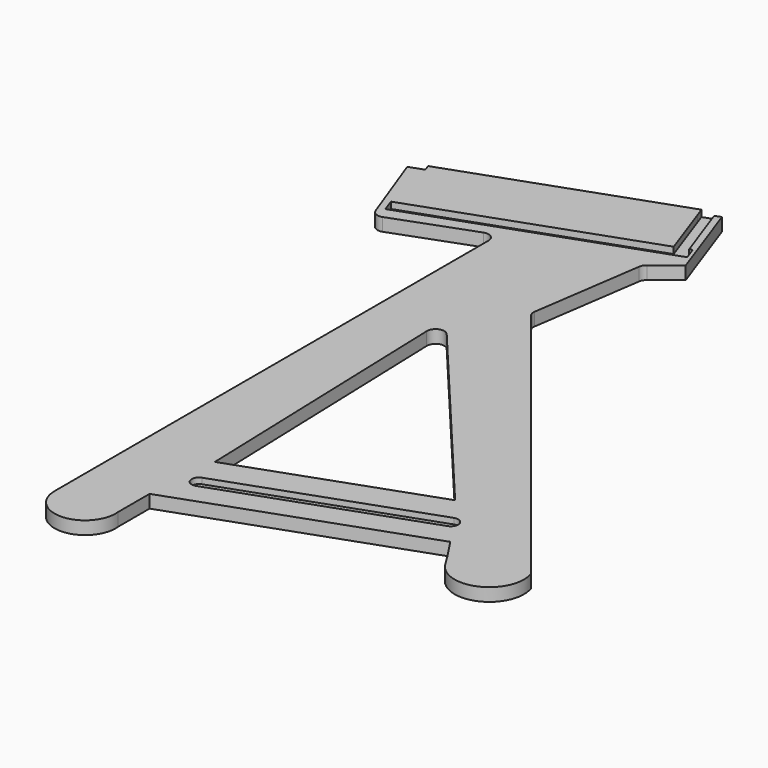
from build123d import *

# Parameters (mm, degrees)
F1_DEPTH = 19.05
F3_DEPTH = 8.4666582
F5_DEPTH = 9.525


# Not quite as in the source:
# - a feature names something its author has since deleted; it is built from what else it names


with BuildPart() as f1:
    # F0 (on Top) → F1 (new body)
    with BuildSketch(Plane.XY):
        with BuildLine():
            Line((727.2677384075, 427.9083177516), (727.2677384075, -283.5772421425))
            ThreePointArc((727.2677384075, -283.5772421425), (774.4074471785, -328.2362889839), (816.4554812019, -278.7535097314))
            Line((816.4554812019, -278.7535097314), (816.4554812019, -221.0955097314))
            Line((816.4554812019, -221.0955097314), (1159.4623036636, -98.9686407408))
            Line((1159.4623036636, -98.9686407408), (1178.6487772739, -128.0367093729))
            Line((1178.6487772739, -128.0367093729), (1189.3036458742, -145.3996676047))
            ThreePointArc((1189.3036458742, -145.3996676047), (1254.3589120262, -165.180351508), (1280.8355912672, -102.5508970465))
            Line((1280.8355912672, -102.5508970465), (881.2480453078, 396.8848219998))
            ThreePointArc((881.2480453078, 396.8848219998), (878.9075846932, 401.4943033077), (878.5980767553, 406.6546597539))
            Line((878.5980767553, 406.6546597539), (902.2401524871, 568.497452094))
            ThreePointArc((902.2401524871, 568.497452094), (903.8120375637, 573.0182606597), (906.9455405898, 576.6362285378))
            Line((906.9455405898, 576.6362285378), (941.9003890149, 604.1852707886))
            Line((941.9003890149, 604.1852707886), (899.3018677789, 723.8279303566))
            Line((899.3018677789, 723.8279303566), (891.7270738587, 721.1309406639))
            Line((891.7270738587, 721.1309406639), (888.532184766, 730.1041401315))
            Line((888.532184766, 730.1041401315), (557.8398737201, 612.361827435))
            Line((557.8398737201, 612.361827435), (561.0347628128, 603.3886279674))
            Line((561.0347628128, 603.3886279674), (540.3738890749, 596.0323666485))
            Line((540.3738890749, 596.0323666485), (579.8650741531, 488.7713005475))
            ThreePointArc((579.8650741531, 488.7713005475), (586.4584656719, 481.6292642269), (596.1708798397, 481.2413137672))
            Line((596.1708798397, 481.2413137672), (710.1798289544, 523.2169221936))
            ThreePointArc((710.1798289544, 523.2169221936), (721.8328450807, 521.7157540947), (727.2677384075, 511.2990259602))
            Line((727.2677384075, 511.2990259602), (727.2677384075, 427.9083177516))
        make_face()
        with BuildLine():
            Line((1099.3852571882, -15.0422832395), (825.3589785984, -112.6087723988))
            Line((825.3589785984, -112.6087723988), (812.2279623998, 291.9047427935))
            ThreePointArc((812.2279623998, 291.9047427935), (820.3847868922, 304.1789193457), (834.6503380579, 300.4798321914))
            Line((834.6503380579, 300.4798321914), (1099.3852571882, -15.0422832395))
        make_face(mode=Mode.SUBTRACT)
    extrude(amount=F1_DEPTH)

    # F2 (on face) → F3 (cut)
    with BuildSketch(Plane.XY.offset(19.05)):
        with BuildLine():
            ThreePointArc((838.451528287, -152.2525984903), (831.9027765287, -166.0430988586), (845.6932768971, -172.5918506169))
            Line((845.6932768971, -172.5918506169), (1132.8356598603, -70.3553996504))
            ThreePointArc((1132.8356598603, -70.3553996504), (1139.3844116185, -56.564899282), (1125.5939112501, -50.0161475238))
            Line((1125.5939112501, -50.0161475238), (838.451528287, -152.2525984903))
        make_face()
    extrude(amount=-F3_DEPTH, mode=Mode.SUBTRACT)

    # F4 (on face) → F5 (cut)
    with BuildSketch(Plane.XY.offset(19.05)):
        Polygon((579.7007303012, 517.0436017545), (586.2609025716, 498.618632181), (926.4367371726, 619.7375338049), (930.6009060633, 621.2201775171), (924.161381266, 639.3062953154), (919.9972123753, 637.8236516032), (891.8491444715, 716.8806143331), (890.4923506062, 720.6913200061), (891.7270738587, 721.1309406639), (888.532184766, 730.1041401315), (869.645537074, 723.3795883228), (874.197220032, 710.5956831823), (902.2246404628, 631.8775722275), align=None)
    extrude(amount=-F5_DEPTH, mode=Mode.SUBTRACT)


solid = f1.part
